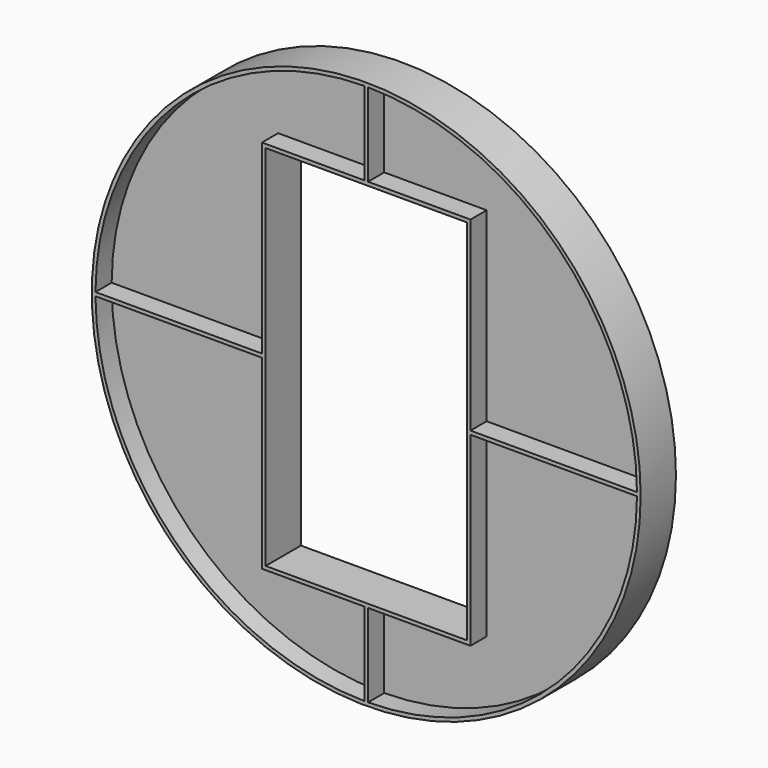
from build123d import *

# Parameters (mm, degrees)
F0_R     = 1897.126
F0_W     = 1390.7516
F0_H     = 2542.9464
F1_DEPTH = 304.8
F2_R     = 1871.726
F2_W     = 1441.5516
F2_H     = 2593.7464
F3_DEPTH = 139.7
F4_R     = 1871.726
F4_W     = 1441.5516
F4_H     = 2593.7464
F5_DEPTH = 139.7
F6_W     = 139.7
F6_H     = 25.4
F9_W     = 25.4
F9_H     = 139.7


# Not quite as in the source:
# - a feature of the source that left no trace in its solid (it failed there, or was rolled back) is left out
# - a pattern or mirror of a feature is missing from the dataset's text; its kind, count and spacing are read off the source's solid


with BuildPart() as f1:
    # F0 (on Front) → F1 (new body)
    with BuildSketch(Plane.XZ):
        Circle(F0_R)
        Rectangle(F0_W, F0_H, mode=Mode.SUBTRACT)
    extrude(amount=F1_DEPTH)

    # F2 (on face) → F3 (cut)
    with BuildSketch(Plane.XZ.offset(304.8)):
        Circle(F2_R)
        Rectangle(F2_W, F2_H, mode=Mode.SUBTRACT)
    extrude(amount=-F3_DEPTH, mode=Mode.SUBTRACT)

    # F4 (on face) → F5 (cut)
    with BuildSketch(Plane(origin=(0, 0, 0), x_dir=(-1, 0, 0), z_dir=(0, 1, 0))):
        Circle(F4_R)
        Rectangle(F4_W, F4_H, mode=Mode.SUBTRACT)
    extrude(amount=-F5_DEPTH, mode=Mode.SUBTRACT)

    # F6 (on face) → F7 (join, up to the next surface of F1)
    with BuildSketch(Plane.YZ.offset(720.7758)):
        with Locations((-234.95, 0)):
            Rectangle(F6_W, F6_H)
    f7 = extrude(until=Until.NEXT)

    # F7_copies: F7 across plane
    add(f7.mirror(Plane.ZX.offset(-152.4)))

    # F8: F1 across plane


with BuildPart() as f1_1:
    add(f1.part)
    add(f1.part.mirror(Plane.YZ))

    # F9 (on face) → F10 (join, up to the next surface of F1)
    with BuildSketch(Plane.XY.offset(1296.8732)):
        with Locations((0, -234.95)):
            Rectangle(F9_W, F9_H)
    extrude(until=Until.NEXT)

    # F11: F1 across plane


with BuildPart() as f1_2:
    add(f1_1.part)
    add(f1_1.part.mirror(Plane.XY))

    # F12 (on face) → F13 (join, up to the next surface of F1)
    with BuildSketch(Plane.XY.offset(1296.8732)):
        Polygon((12.6997518255, -139.6206049634), (12.5756783059, 0), (-12.823825345, -0.1587900733), (-12.6997518255, -139.7793950366), align=None)
    extrude(until=Until.NEXT)

    # F14: F1 across plane


with BuildPart() as f1_3:
    add(f1_2.part)
    add(f1_2.part.mirror(Plane.XY))


solid = f1_3.part
